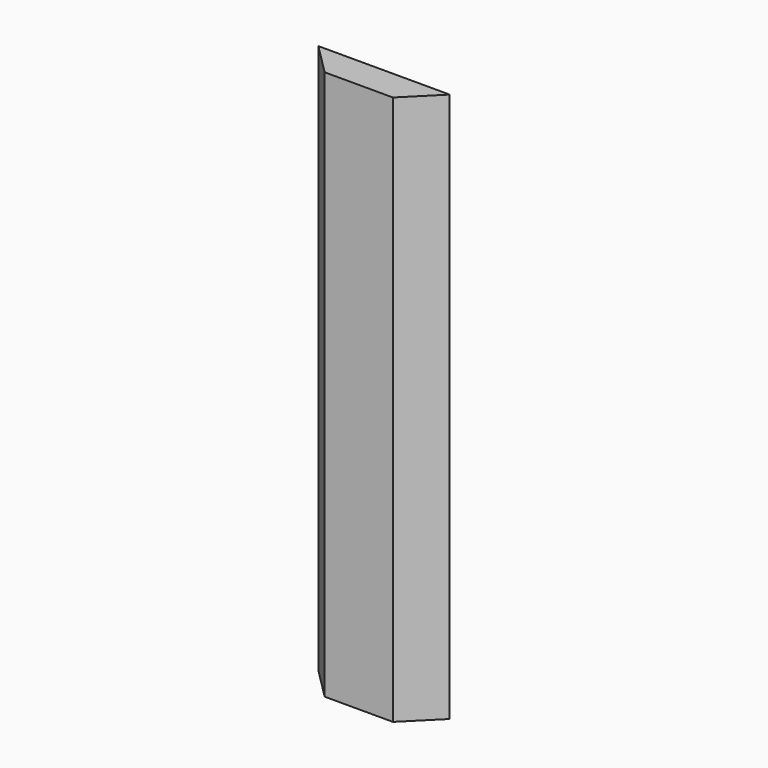
from build123d import *

# Parameters (mm, degrees)
F0_W     = 75
F0_H     = 314
F1_DEPTH = 18
F2_SIZE  = 17.99999


# Not quite as in the source:
# - a fillet or chamfer is up to 0.001 mm smaller than in the source, because OpenCascade refuses the exact size


with BuildPart() as f1:
    # F0 (on Front) → F1 (new body)
    with BuildSketch(Plane.XZ):
        Rectangle(F0_W, F0_H)
    extrude(amount=F1_DEPTH)

    # F2 (size 18 in the source; OpenCascade refuses exactly that, so slightly less here)
    f2_edges = [f1.edges().sort_by_distance(p)[0] for p in [
        (37.5, -18, 0),
        (-37.5, -18, 0),
    ]]
    chamfer(f2_edges, length=F2_SIZE)


solid = f1.part
